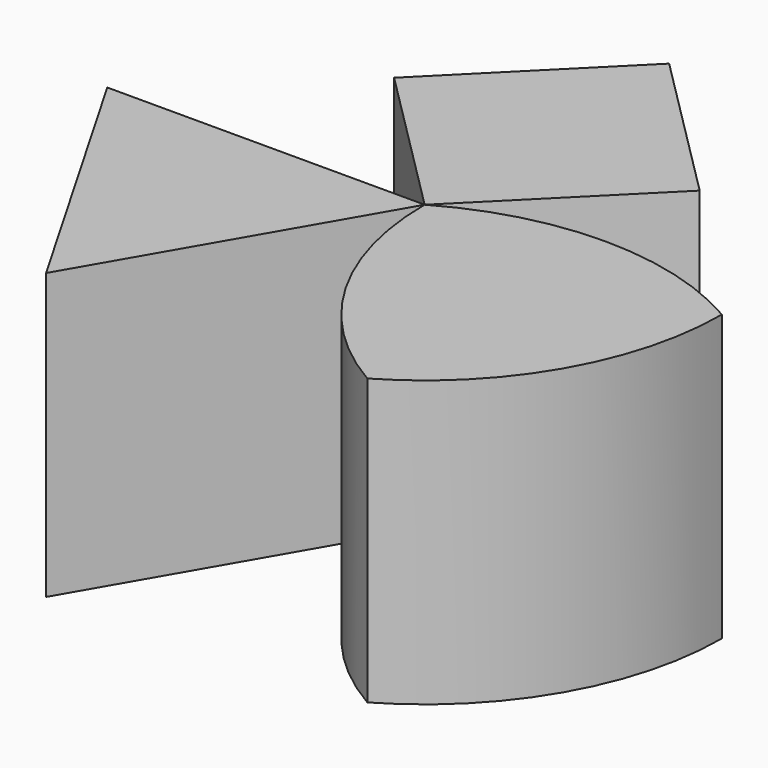
from build123d import *

# Parameters (mm, degrees)
F1_DEPTH = 25.4
F3_DEPTH = 25.4
F5_DEPTH = 25.4


with BuildPart() as f1:
    # F0 (on Top) → F1 (new body)
    with BuildSketch(Plane.XY):
        Polygon((0, 0), (-28.2685179263, 0), (-14.1342589632, -24.4812546515), align=None)
    extrude(amount=F1_DEPTH)


with BuildPart() as f3:
    # F2 (on Top) → F3 (new body)
    with BuildSketch(Plane.XY):
        with BuildLine():
            ThreePointArc((13.2381515749, -22.9291511259), (22.9291511259, -13.2381515749), (26.4763031497, 0))
            ThreePointArc((26.4763031497, 0), (13.2381515749, 3.5471520238), (0, 0))
            ThreePointArc((0, 0), (3.5471520238, -13.2381515749), (13.2381515749, -22.9291511259))
        make_face()
    extrude(amount=F3_DEPTH)


with BuildPart() as f5:
    # F4 (on Top) → F5 (new body)
    with BuildSketch(Plane.XY):
        Polygon((13.6095220223, 13.6095220223), (0, 27.2190440446), (-13.6095220223, 13.6095220223), (0, 0), align=None)
    extrude(amount=F5_DEPTH)


solid = Compound([f1.part, f3.part, f5.part])
